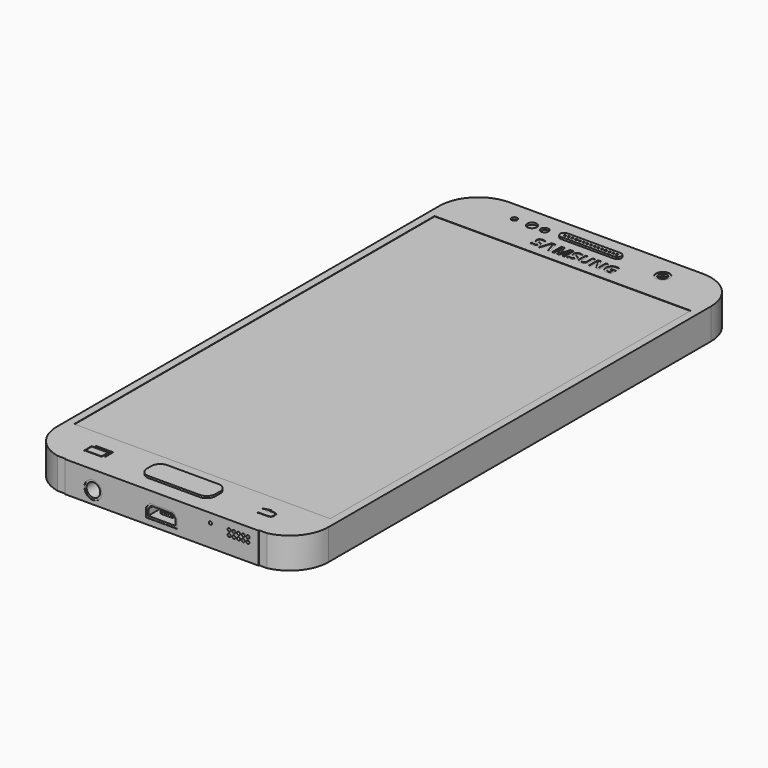
from build123d import *

# Parameters (mm, degrees)
F0_W          = 69.6
F0_H          = 142.4
F1_DEPTH      = 7.9
F2_R          = 10
F4_W          = 17.6
F4_H          = 6
F5_DEPTH      = 0.5
F6_R          = 2.25
F3_W          = 65.6
F3_H          = 115.4
F7_DEPTH      = 0.1
F8_W          = 15.6
F8_H          = 2
F9_DEPTH      = 0.5
F10_R         = 0.99999
F11_R         = 1
F11_R_2       = 1.25
F11_R_3       = 0.75
F12_DEPTH     = 0.5
F13_R         = 0.25
F14_DEPTH     = 3
F15_R         = 1.75
F16_DEPTH     = 0.1
F17_R         = 1.125
F18_DEPTH     = 0.5
F19_R         = 0.5
F20_DEPTH     = 0.1
F21_TEXT_SIZE = 4.1666666667
F22_DEPTH     = 0.1
F24_DEPTH     = 0.1
F25_W         = 4.6
F25_H         = 2.525
F25_W_2       = 4
F25_H_2       = 1.925
F26_DEPTH     = 0.1
F28_DEPTH     = 0.1
F29_R         = 2.25
F30_DEPTH     = 0.1
F31_R         = 1.75
F32_DEPTH     = 10
F33_W         = 2
F33_H         = 7.9
F34_DEPTH     = 0.2
F36_DEPTH     = 0.1
F38_DEPTH     = 4
F40_DEPTH     = 2.5
F41_R         = 0.4
F42_DEPTH     = 10


# Not quite as in the source:
# - a fillet or chamfer is up to 0.001 mm smaller than in the source, because OpenCascade refuses the exact size
# - Text() gives the source's letters only with a copy of the font that has no kerning and outlines rounded to 1/6400 em; it was checked with that copy


with BuildPart() as f1:
    # F0 (on Top) → F1 (new body)
    with BuildSketch(Plane.XY):
        with Locations((34.8, -71.2)):
            Rectangle(F0_W, F0_H)
    extrude(amount=F1_DEPTH)

    # F2
    f2_edges = [f1.edges().sort_by_distance(p)[0] for p in [
        (69.6, -142.4, 3.95),
        (0, -142.4, 3.95),
        (69.6, 0, 3.95),
        (0, 0, 3.95),
    ]]
    fillet(f2_edges, radius=F2_R)

    # F4 (on face) → F5 (join)
    with BuildSketch(Plane.XY.offset(7.9)):
        with Locations((34.8, -135.4)):
            Rectangle(F4_W, F4_H)
    extrude(amount=F5_DEPTH)

    # F6
    f6_edges = [f1.edges().sort_by_distance(p)[0] for p in [
        (26, -132.4, 8.15),
        (43.6, -132.4, 8.15),
        (26, -138.4, 8.15),
        (43.6, -138.4, 8.15),
    ]]
    fillet(f6_edges, radius=F6_R)

    # F3 (on face) → F7 (cut)
    with BuildSketch(Plane.XY.offset(7.9)):
        with Locations((34.8, -71.7)):
            Rectangle(F3_W, F3_H)
    extrude(amount=-F7_DEPTH, mode=Mode.SUBTRACT)

    # F8 (on face) → F9 (join)
    with BuildSketch(Plane.XY.offset(7.9)):
        with Locations((34.8, -5)):
            Rectangle(F8_W, F8_H)
    extrude(amount=F9_DEPTH)

    # F10 (radius 1 in the source; OpenCascade refuses exactly that, so slightly less here)
    f10_edges = [f1.edges().sort_by_distance(p)[0] for p in [
        (42.6, -4, 8.15),
        (27, -4, 8.15),
        (42.6, -6, 8.15),
        (27, -6, 8.15),
    ]]
    fillet(f10_edges, radius=F10_R)

    # F11 (on face) → F12 (cut)
    with BuildSketch(Plane.XY.offset(7.9)):
        with Locations((23, -5)):
            Circle(F11_R)
        with Locations((19.75, -5)):
            Circle(F11_R_2)
        with Locations((15.25, -5)):
            Circle(F11_R_3)
    extrude(amount=-F12_DEPTH, mode=Mode.SUBTRACT)

    # F13 (on face) → F14 (cut)
    with BuildSketch(Plane.XY.offset(8.4)):
        with Locations((28.2, -5)):
            Circle(F13_R)
        with Locations((29.15, -5)):
            Circle(F13_R)
        with Locations((30.1, -5)):
            Circle(F13_R)
        with Locations((31.05, -5)):
            Circle(F13_R)
        with Locations((32, -5)):
            Circle(F13_R)
        with Locations((32.95, -5)):
            Circle(F13_R)
        with Locations((33.9, -5)):
            Circle(F13_R)
        with Locations((34.85, -5)):
            Circle(F13_R)
        with Locations((35.8, -5)):
            Circle(F13_R)
        with Locations((36.75, -5)):
            Circle(F13_R)
        with Locations((37.7, -5)):
            Circle(F13_R)
        with Locations((38.65, -5)):
            Circle(F13_R)
        with Locations((39.6, -5)):
            Circle(F13_R)
        with Locations((40.55, -5)):
            Circle(F13_R)
        with Locations((41.5, -5)):
            Circle(F13_R)
    extrude(amount=-F14_DEPTH, mode=Mode.SUBTRACT)

    # F15 (on face) → F16 (cut)
    with BuildSketch(Plane.XY.offset(7.9)):
        with Locations((53.85, -5.75)):
            Circle(F15_R)
    extrude(amount=-F16_DEPTH, mode=Mode.SUBTRACT)

    # F17 (on face) → F18 (cut)
    with BuildSketch(Plane.XY.offset(7.8)):
        with Locations((53.85, -5.75)):
            Circle(F17_R)
    extrude(amount=-F18_DEPTH, mode=Mode.SUBTRACT)

    # F19 (on face) → F20 (cut)
    with BuildSketch(Plane.XY.offset(7.3)):
        with Locations((53.85, -5.75)):
            Circle(F19_R)
    extrude(amount=-F20_DEPTH, mode=Mode.SUBTRACT)

    # F21 (on face) → F22 (cut)
    with BuildSketch(Plane.XY.offset(7.9)):
        with Locations((24.1714192708, -11.5)):
            Text('S   MSUNG', F21_TEXT_SIZE, font='Open Sans', font_style=FontStyle.BOLD, text_align=(TextAlign.LEFT, TextAlign.BOTTOM))
    extrude(amount=-F22_DEPTH, mode=Mode.SUBTRACT)

    # F23 (on face) → F24 (cut)
    with BuildSketch(Plane.XY.offset(7.9)):
        Polygon((28.6222278046, -8.525390625), (27.6681367787, -8.525390625), (26.7016276042, -11.5), (27.2797526042, -11.5), (28.1451822917, -8.8364812982), (29.0106119792, -11.5), (29.5887369792, -11.5), align=None)
    extrude(amount=-F24_DEPTH, mode=Mode.SUBTRACT)

    # F25 (on face) → F26 (cut)
    with BuildSketch(Plane.XY.offset(7.9)):
        with Locations((13, -135.9125)):
            Rectangle(F25_W, F25_H)
        with Locations((13, -135.9125)):
            Rectangle(F25_W_2, F25_H_2, mode=Mode.SUBTRACT)
        Polygon((15.9, -134.05), (11.3, -134.05), (11.3, -134.35), (15.6, -134.35), (15.6, -136.575), (15.9, -136.575), align=None)
    extrude(amount=-F26_DEPTH, mode=Mode.SUBTRACT)

    # F27 (on face) → F28 (cut)
    with BuildSketch(Plane.XY.offset(7.9)):
        with BuildLine():
            Line((57.1, -136.25), (54.6, -136.25))
            Line((54.6, -136.25), (54.6, -136.55))
            Line((54.6, -136.55), (57.1, -136.55))
            ThreePointArc((57.1, -136.55), (58.25, -135.4), (57.1, -134.25))
            Line((57.1, -134.25), (56.1, -134.25))
            Line((56.1, -134.25), (56.1, -133.85))
            Line((56.1, -133.85), (54.1, -134.4))
            Line((54.1, -134.4), (56.1, -134.95))
            Line((56.1, -134.95), (56.1, -134.55))
            Line((56.1, -134.55), (57.1, -134.55))
            ThreePointArc((57.1, -134.55), (57.95, -135.4), (57.1, -136.25))
        make_face()
    extrude(amount=-F28_DEPTH, mode=Mode.SUBTRACT)

    # F29 (on face) → F30 (cut)
    with BuildSketch(Plane.XZ.offset(142.4)):
        with Locations((17.25, 3.25)):
            Circle(F29_R)
    extrude(amount=-F30_DEPTH, mode=Mode.SUBTRACT)

    # F31 (on face) → F32 (cut)
    with BuildSketch(Plane.XZ.offset(142.3)):
        with Locations((17.25, 3.25)):
            Circle(F31_R)
    extrude(amount=-F32_DEPTH, mode=Mode.SUBTRACT)

    # F33 (on face) → F34 (cut)
    with BuildSketch(Plane.XZ.offset(142.4)):
        with Locations((9, 3.95)):
            Rectangle(F33_W, F33_H)
        with Locations((60.6, 3.95)):
            Rectangle(F33_W, F33_H)
    extrude(amount=-F34_DEPTH, mode=Mode.SUBTRACT)

    # F35 (on face) → F36 (cut)
    with BuildSketch(Plane.XZ.offset(142.4)):
        Polygon((30.8, 3.75), (30.8, 1.5), (38.8, 1.5), (38.8, 3.75), (37.8, 5), (31.8, 5), align=None)
    extrude(amount=-F36_DEPTH, mode=Mode.SUBTRACT)

    # F37 (on face) → F38 (cut)
    with BuildSketch(Plane.XZ.offset(142.3)):
        Polygon((31.3, 3.5746094703), (31.3, 2), (38.3, 2), (38.3, 3.5746094703), (37.5596875763, 4.5), (32.0403124237, 4.5), align=None)
    extrude(amount=-F38_DEPTH, mode=Mode.SUBTRACT)

    # F39 (on face) → F40 (join)
    with BuildSketch(Plane.XZ.offset(138.3)):
        Polygon((33.3, 3.2), (33.3, 2.5), (36.3, 2.5), (36.3, 3.2), (36.02, 3.2), (36.02, 2.95), (35.756, 2.95), (35.756, 3.2), (35.476, 3.2), (35.476, 2.95), (35.212, 2.95), (35.212, 3.2), (34.932, 3.2), (34.932, 2.95), (34.668, 2.95), (34.668, 3.2), (34.388, 3.2), (34.388, 2.95), (34.124, 2.95), (34.124, 3.2), (33.844, 3.2), (33.844, 2.95), (33.58, 2.95), (33.58, 3.2), align=None)
    extrude(amount=F40_DEPTH)

    # F41 (on face) → F42 (cut)
    with BuildSketch(Plane.XZ.offset(142.4)):
        with Locations((56.9, 5.6044650264)):
            Circle(F41_R)
        with Locations((56.9, 4.4044650264)):
            Circle(F41_R)
        with Locations((55.7, 5.6044650264)):
            Circle(F41_R)
        with Locations((55.7, 4.4044650264)):
            Circle(F41_R)
        with Locations((54.5, 5.6044650264)):
            Circle(F41_R)
        with Locations((54.5, 4.4044650264)):
            Circle(F41_R)
        with Locations((53.3, 5.6044650264)):
            Circle(F41_R)
        with Locations((53.3, 4.4044650264)):
            Circle(F41_R)
        with Locations((52.1, 5.6044650264)):
            Circle(F41_R)
        with Locations((52.1, 4.4044650264)):
            Circle(F41_R)
        with Locations((47.3, 5.6044650264)):
            Circle(F41_R)
    extrude(amount=-F42_DEPTH, mode=Mode.SUBTRACT)


solid = f1.part
